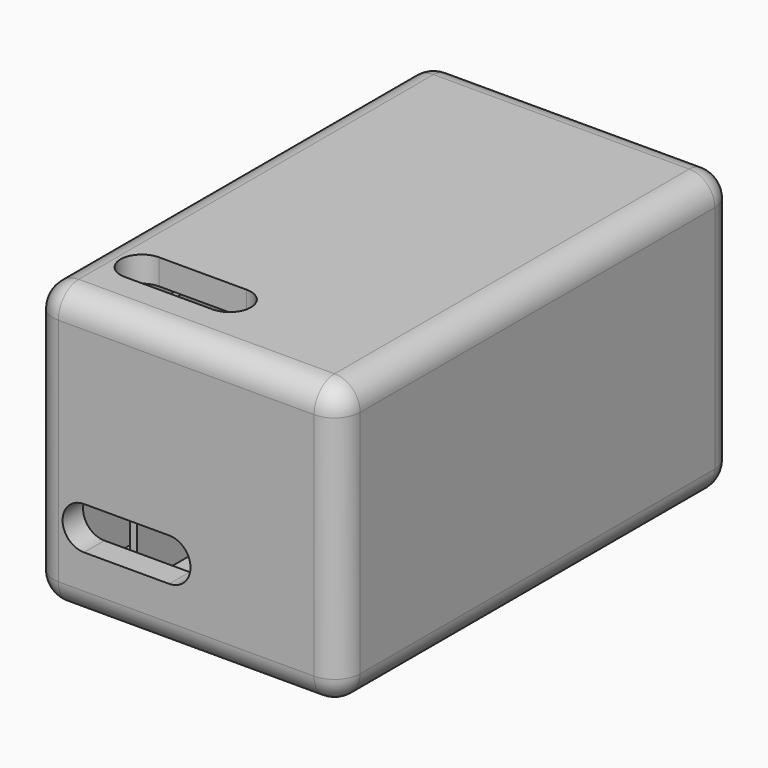
from build123d import *

# Parameters (mm, degrees)
F0_W      = 36
F0_H      = 58
F0_W_2    = 30
F0_H_2    = 52
F1_DEPTH  = 30
F2_DEPTH  = 2.5
F3_W      = 10
F3_H      = 5
F4_DEPTH  = 25
F5_START  = 30
F5_DEPTH  = 3
F6_R      = 2.99999
F6_2_R    = 2.99999
F7_W      = 10.2862860618
F7_H      = 5
F8_DEPTH  = 3
F9_W      = 0.8
F9_H      = 49
F10_DEPTH = 27.5


# Not quite as in the source:
# - a fillet or chamfer is up to 0.001 mm smaller than in the source, because OpenCascade refuses the exact size


with BuildPart() as f1:
    # F0 (on Top) → F1 (new body)
    with BuildSketch(Plane.XY):
        Rectangle(F0_W, F0_H)
        Rectangle(F0_W_2, F0_H_2, mode=Mode.SUBTRACT)
    extrude(amount=F1_DEPTH)

    # F0 (on Top) → F2 (join)
    with BuildSketch(Plane.XY):
        Rectangle(F0_W_2, F0_H_2)
    extrude(amount=F2_DEPTH)

    # F3 (on face) → F4 (cut)
    with BuildSketch(Plane.XZ.offset(29)):
        with Locations((-7, 9.5)):
            Rectangle(F3_W, F3_H)
        with BuildLine():
            Line((-12, 7), (-12, 12))
            ThreePointArc((-12, 12), (-14.5, 9.5), (-12, 7))
        make_face()
        with BuildLine():
            ThreePointArc((-2, 7), (0.5, 9.5), (-2, 12))
            Line((-2, 12), (-2, 7))
        make_face()
    extrude(amount=-F4_DEPTH, mode=Mode.SUBTRACT)

    # F6 (radius 3 in the source; OpenCascade refuses exactly that, so slightly less here)
    f6_edges = [f1.edges().sort_by_distance(p)[0] for p in [
        (0, 29, 0),
        (-18, 0, 0),
        (0, -29, 0),
        (18, 0, 0),
        (-18, -29, 15),
        (18, -29, 15),
        (18, 29, 15),
        (-18, 29, 15),
    ]]
    fillet(f6_edges, radius=F6_R)

    # F9 (on face) → F10 (join)
    with BuildSketch(Plane.XY.offset(2.5)):
        with Locations((-9.8, 0)):
            Rectangle(F9_W, F9_H)
        Rectangle(F9_W, F9_H)
        with Locations((9.8, 0)):
            Rectangle(F9_W, F9_H)
    extrude(amount=F10_DEPTH)


with BuildPart() as f5:
    # F0 (on Top) → F5 (new body)
    with BuildSketch(Plane.XY.offset(F5_START)):
        Rectangle(F0_W, F0_H)
        Rectangle(F0_W_2, F0_H_2, mode=Mode.SUBTRACT)
        Rectangle(F0_W_2, F0_H_2)
    extrude(amount=F5_DEPTH)

    # F6#2 (radius 3 in the source; OpenCascade refuses exactly that, so slightly less here)
    f6_2_edges = [f5.edges().sort_by_distance(p)[0] for p in [
        (-18, -29, 31.5),
        (0, 29, 33),
        (-18, 0, 33),
        (0, -29, 33),
        (18, 0, 33),
        (18, -29, 31.5),
        (18, 29, 31.5),
        (-18, 29, 31.5),
    ]]
    fillet(f6_2_edges, radius=F6_2_R)

    # F7 (on face) → F8 (cut)
    with BuildSketch(Plane.XY.offset(33)):
        with Locations((-6.8568569691, -20.5)):
            Rectangle(F7_W, F7_H)
        with BuildLine():
            Line((-12, -23), (-12, -18))
            ThreePointArc((-12, -18), (-14.5, -20.5), (-12, -23))
        make_face()
        with BuildLine():
            ThreePointArc((-1.7137139382, -23), (0.7862860618, -20.5), (-1.7137139382, -18))
            Line((-1.7137139382, -18), (-1.7137139382, -23))
        make_face()
    extrude(amount=-F8_DEPTH, mode=Mode.SUBTRACT)


solid = Compound([f1.part, f5.part])
